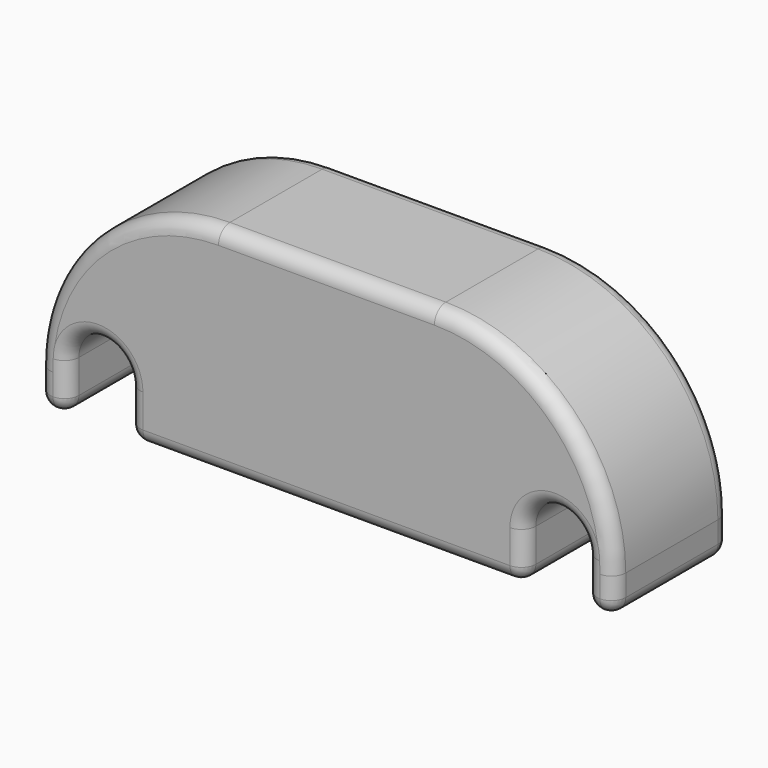
from build123d import *

# Parameters (mm, degrees)
F1_DEPTH     = 20
F2_R         = 1.99999
F3_T1_DEPTH  = 30
F3_T3_DEPTH  = 8.00001
F3_T5_DEPTH  = 10.00002
F3_T7_DEPTH  = 9.6446849121
F3_T9_DEPTH  = 61.00002
F3_T11_DEPTH = 10.00002
F3_T14_ANGLE = 90
F3_T16_ANGLE = 90
F3_T18_ANGLE = 90
F3_T20_ANGLE = 90
F3_T22_ANGLE = 180
F3_T24_ANGLE = 90
F3_T26_ANGLE = 90
F3_T28_ANGLE = 180
F3_T30_ANGLE = 90
F3_T32_ANGLE = 90
F3_T34_ANGLE = 90
F3_T36_ANGLE = 90
F3_T38_ANGLE = 90
F3_T40_ANGLE = 90
F3_T42_ANGLE = 180
F3_T44_ANGLE = 90
F3_T46_ANGLE = 90
F3_T48_ANGLE = 180
F3_T50_ANGLE = 90
F3_T52_ANGLE = 90


# Not quite as in the source:
# - a fillet or chamfer that OpenCascade refuses, or shapes differently, is made with other operations: its cross-section is extruded or revolved along the edge and cut away or added
# - a fillet or chamfer is up to 0.001 mm smaller than in the source, because OpenCascade refuses the exact size


with BuildPart() as f1:
    # F0 (on Front) → F1 (new body)
    with BuildSketch(Plane.XZ):
        with BuildLine():
            Line((15, 15), (-15, 15))
            ThreePointArc((-15, 15), (-32.6776695297, 7.6776695297), (-40, -10))
            Line((-40, -10), (-40, -15))
            Line((-40, -15), (-36, -15))
            Line((-36, -15), (-36, -8.3553250879))
            ThreePointArc((-36, -8.3553250879), (-31.75, -4.1053250879), (-27.5, -8.3553250879))
            Line((-27.5, -8.3553250879), (-27.5, -15))
            Line((-27.5, -15), (27.5, -15))
            Line((27.5, -15), (27.5, -8.3553250879))
            ThreePointArc((27.5, -8.3553250879), (31.75, -4.1053250879), (36, -8.3553250879))
            Line((36, -8.3553250879), (36, -15))
            Line((36, -15), (40, -15))
            Line((40, -15), (40, -10))
            ThreePointArc((40, -10), (32.6776695297, 7.6776695297), (15, 15))
        make_face()
    extrude(amount=F1_DEPTH)

    # F2 (radius 2 in the source; OpenCascade refuses exactly that, so slightly less here)
    f2_edges = [f1.edges().sort_by_distance(p)[0] for p in [
        (36, -10, -15),
        (27.5, -10, -15),
        (40, -10, -15),
        (-27.5, -10, -15),
        (-36, -10, -15),
        (-40, -10, -15),
    ]]
    fillet(f2_edges, radius=F2_R)

    # F3: fillet of radius 2 on 2 edges, made by hand

    # F3_s2 → F3_t1 (cut)
    with BuildSketch(Plane.YZ.offset(-15)):
        with BuildLine():
            ThreePointArc((0, 13), (-0.5857864376, 14.4142135624), (-2, 15))
            Line((-2, 15), (0, 15))
            Line((0, 15), (0, 13))
        make_face()
        with BuildLine():
            ThreePointArc((-20, 13), (-19.4142135624, 14.4142135624), (-18, 15))
            Line((-18, 15), (-20, 15))
            Line((-20, 15), (-20, 13))
        make_face()
    extrude(amount=F3_T1_DEPTH, mode=Mode.SUBTRACT)

    # F3_s4 → F3_t3 (cut)
    with BuildSketch(Plane.XY.offset(-18.00001)):
        with BuildLine():
            ThreePointArc((38, -20), (39.4142135624, -19.4142135624), (40, -18))
            Line((40, -18), (40, -20))
            Line((40, -20), (38, -20))
        make_face()
        with BuildLine():
            ThreePointArc((-40, -18), (-39.4142135624, -19.4142135624), (-38, -20))
            Line((-38, -20), (-40, -20))
            Line((-40, -20), (-40, -18))
        make_face()
        with BuildLine():
            ThreePointArc((-40, -2), (-39.4142135624, -0.5857864376), (-38, 0))
            Line((-38, 0), (-40, 0))
            Line((-40, 0), (-40, -2))
        make_face()
        with BuildLine():
            ThreePointArc((38, 0), (39.4142135624, -0.5857864376), (40, -2))
            Line((40, -2), (40, 0))
            Line((40, 0), (38, 0))
        make_face()
    extrude(amount=F3_T3_DEPTH, mode=Mode.SUBTRACT)

    # F3_s6 → F3_t5 (cut)
    with BuildSketch(Plane.YZ.offset(-43.00001)):
        with BuildLine():
            ThreePointArc((-20, -13), (-19.4142135624, -14.4142135624), (-18, -15))
            Line((-18, -15), (-20, -15))
            Line((-20, -15), (-20, -13))
        make_face()
        with BuildLine():
            ThreePointArc((0, -13), (-0.5857864376, -14.4142135624), (-2, -15))
            Line((-2, -15), (0, -15))
            Line((0, -15), (0, -13))
        make_face()
    extrude(amount=F3_T5_DEPTH, mode=Mode.SUBTRACT)

    # F3_s8 → F3_t7 (cut)
    with BuildSketch(Plane.XY.offset(-18.00001)):
        with BuildLine():
            ThreePointArc((-38, -20), (-36.5857864376, -19.4142135624), (-36, -18))
            Line((-36, -18), (-36, -20))
            Line((-36, -20), (-38, -20))
        make_face()
        with BuildLine():
            ThreePointArc((-25.5, -20), (-26.9142135624, -19.4142135624), (-27.5, -18))
            Line((-27.5, -18), (-27.5, -20))
            Line((-27.5, -20), (-25.5, -20))
        make_face()
        with BuildLine():
            ThreePointArc((25.5, -20), (26.9142135624, -19.4142135624), (27.5, -18))
            Line((27.5, -18), (27.5, -20))
            Line((27.5, -20), (25.5, -20))
        make_face()
        with BuildLine():
            ThreePointArc((38, -20), (36.5857864376, -19.4142135624), (36, -18))
            Line((36, -18), (36, -20))
            Line((36, -20), (38, -20))
        make_face()
        with BuildLine():
            ThreePointArc((-38, 0), (-36.5857864376, -0.5857864376), (-36, -2))
            Line((-36, -2), (-36, 0))
            Line((-36, 0), (-38, 0))
        make_face()
        with BuildLine():
            ThreePointArc((-25.5, 0), (-26.9142135624, -0.5857864376), (-27.5, -2))
            Line((-27.5, -2), (-27.5, 0))
            Line((-27.5, 0), (-25.5, 0))
        make_face()
        with BuildLine():
            ThreePointArc((25.5, 0), (26.9142135624, -0.5857864376), (27.5, -2))
            Line((27.5, -2), (27.5, 0))
            Line((27.5, 0), (25.5, 0))
        make_face()
        with BuildLine():
            ThreePointArc((38, 0), (36.5857864376, -0.5857864376), (36, -2))
            Line((36, -2), (36, 0))
            Line((36, 0), (38, 0))
        make_face()
    extrude(amount=F3_T7_DEPTH, mode=Mode.SUBTRACT)

    # F3_s10 → F3_t9 (cut)
    with BuildSketch(Plane.YZ.offset(-30.50001)):
        with BuildLine():
            ThreePointArc((-20, -13), (-19.4142135624, -14.4142135624), (-18, -15))
            Line((-18, -15), (-20, -15))
            Line((-20, -15), (-20, -13))
        make_face()
        with BuildLine():
            ThreePointArc((0, -13), (-0.5857864376, -14.4142135624), (-2, -15))
            Line((-2, -15), (0, -15))
            Line((0, -15), (0, -13))
        make_face()
    extrude(amount=F3_T9_DEPTH, mode=Mode.SUBTRACT)

    # F3_s12 → F3_t11 (cut)
    with BuildSketch(Plane.YZ.offset(32.99999)):
        with BuildLine():
            ThreePointArc((-20, -13), (-19.4142135624, -14.4142135624), (-18, -15))
            Line((-18, -15), (-20, -15))
            Line((-20, -15), (-20, -13))
        make_face()
        with BuildLine():
            ThreePointArc((0, -13), (-0.5857864376, -14.4142135624), (-2, -15))
            Line((-2, -15), (0, -15))
            Line((0, -15), (0, -13))
        make_face()
    extrude(amount=F3_T11_DEPTH, mode=Mode.SUBTRACT)

    # F3_s13 → F3_t14 (revolve, cut)
    with BuildSketch(Plane.XY.offset(-10)):
        with BuildLine():
            ThreePointArc((38, -20), (39.4142135624, -19.4142135624), (40, -18))
            Line((40, -18), (40, -20))
            Line((40, -20), (38, -20))
        make_face()
    revolve(axis=Axis((15, -20, -10), (0, -1, 0)), revolution_arc=F3_T14_ANGLE, mode=Mode.SUBTRACT)

    # F3_s15 → F3_t16 (revolve, cut)
    with BuildSketch(Plane.YZ.offset(-15)):
        with BuildLine():
            ThreePointArc((-18, 15), (-19.4142135624, 14.4142135624), (-20, 13))
            Line((-20, 13), (-20, 15))
            Line((-20, 15), (-18, 15))
        make_face()
    revolve(axis=Axis((-15, -20, -10), (0, -1, 0)), revolution_arc=F3_T16_ANGLE, mode=Mode.SUBTRACT)

    # F3_s17 → F3_t18 (revolve, cut)
    with BuildSketch(Plane.XY.offset(-13.00001)):
        with BuildLine():
            ThreePointArc((-40, -18), (-39.4142170979, -19.4142100268), (-38.00001, -20))
            Line((-38.00001, -20), (-40, -20))
            Line((-40, -20), (-40, -18))
        make_face()
    revolve(axis=Axis((-38.00001, -20, -13.00001), (0, -1, 0)), revolution_arc=F3_T18_ANGLE, mode=Mode.SUBTRACT)

    # F3_s19 → F3_t20 (revolve, cut)
    with BuildSketch(Plane.YZ.offset(-37.99999)):
        with BuildLine():
            ThreePointArc((-20, -13.00001), (-19.4142100268, -14.4142170979), (-18, -15))
            Line((-18, -15), (-20, -15))
            Line((-20, -15), (-20, -13.00001))
        make_face()
    revolve(axis=Axis((-37.99999, -20, -13.00001), (0, -1, 0)), revolution_arc=F3_T20_ANGLE, mode=Mode.SUBTRACT)

    # F3_s21 → F3_t22 (revolve, cut)
    with BuildSketch(Plane.XY.offset(-8.3553250879)):
        with BuildLine():
            ThreePointArc((-38, -20), (-36.5857864376, -19.4142135624), (-36, -18))
            Line((-36, -18), (-36, -20))
            Line((-36, -20), (-38, -20))
        make_face()
    revolve(axis=Axis((-31.75, -20, -8.3553250879), (0, 1, 0)), revolution_arc=F3_T22_ANGLE, mode=Mode.SUBTRACT)

    # F3_s23 → F3_t24 (revolve, cut)
    with BuildSketch(Plane.XY.offset(-13.00001)):
        with BuildLine():
            ThreePointArc((-25.50001, -20), (-26.9142170979, -19.4142100268), (-27.5, -18))
            Line((-27.5, -18), (-27.5, -20))
            Line((-27.5, -20), (-25.50001, -20))
        make_face()
    revolve(axis=Axis((-25.50001, -20, -13.00001), (0, -1, 0)), revolution_arc=F3_T24_ANGLE, mode=Mode.SUBTRACT)

    # F3_s25 → F3_t26 (revolve, cut)
    with BuildSketch(Plane.YZ.offset(25.50001)):
        with BuildLine():
            ThreePointArc((-20, -13.00001), (-19.4142100268, -14.4142170979), (-18, -15))
            Line((-18, -15), (-20, -15))
            Line((-20, -15), (-20, -13.00001))
        make_face()
    revolve(axis=Axis((25.50001, -20, -13.00001), (0, -1, 0)), revolution_arc=F3_T26_ANGLE, mode=Mode.SUBTRACT)

    # F3_s27 → F3_t28 (revolve, cut)
    with BuildSketch(Plane.XY.offset(-8.3553250879)):
        with BuildLine():
            ThreePointArc((25.5, -20), (26.9142135624, -19.4142135624), (27.5, -18))
            Line((27.5, -18), (27.5, -20))
            Line((27.5, -20), (25.5, -20))
        make_face()
    revolve(axis=Axis((31.75, -20, -8.3553250879), (0, 1, 0)), revolution_arc=F3_T28_ANGLE, mode=Mode.SUBTRACT)

    # F3_s29 → F3_t30 (revolve, cut)
    with BuildSketch(Plane.XY.offset(-13.00001)):
        with BuildLine():
            ThreePointArc((37.99999, -20), (36.5857829021, -19.4142100268), (36, -18))
            Line((36, -18), (36, -20))
            Line((36, -20), (37.99999, -20))
        make_face()
    revolve(axis=Axis((37.99999, -20, -13.00001), (0, -1, 0)), revolution_arc=F3_T30_ANGLE, mode=Mode.SUBTRACT)

    # F3_s31 → F3_t32 (revolve, cut)
    with BuildSketch(Plane.YZ.offset(38.00001)):
        with BuildLine():
            ThreePointArc((-20, -13.00001), (-19.4142100268, -14.4142170979), (-18, -15))
            Line((-18, -15), (-20, -15))
            Line((-20, -15), (-20, -13.00001))
        make_face()
    revolve(axis=Axis((38.00001, -20, -13.00001), (0, -1, 0)), revolution_arc=F3_T32_ANGLE, mode=Mode.SUBTRACT)

    # F3_s33 → F3_t34 (revolve, cut)
    with BuildSketch(Plane.XY.offset(-10)):
        with BuildLine():
            ThreePointArc((38, 0), (39.4142135624, -0.5857864376), (40, -2))
            Line((40, -2), (40, 0))
            Line((40, 0), (38, 0))
        make_face()
    revolve(axis=Axis((15, 0, -10), (0, -1, 0)), revolution_arc=F3_T34_ANGLE, mode=Mode.SUBTRACT)

    # F3_s35 → F3_t36 (revolve, cut)
    with BuildSketch(Plane.YZ.offset(-15)):
        with BuildLine():
            ThreePointArc((0, 13), (-0.5857864376, 14.4142135624), (-2, 15))
            Line((-2, 15), (0, 15))
            Line((0, 15), (0, 13))
        make_face()
    revolve(axis=Axis((-15, 0, -10), (0, -1, 0)), revolution_arc=F3_T36_ANGLE, mode=Mode.SUBTRACT)

    # F3_s37 → F3_t38 (revolve, cut)
    with BuildSketch(Plane.XY.offset(-13.00001)):
        with BuildLine():
            ThreePointArc((-38.00001, 0), (-39.4142170979, -0.5857899732), (-40, -2))
            Line((-40, -2), (-40, 0))
            Line((-40, 0), (-38.00001, 0))
        make_face()
    revolve(axis=Axis((-38.00001, 0, -13.00001), (0, -1, 0)), revolution_arc=F3_T38_ANGLE, mode=Mode.SUBTRACT)

    # F3_s39 → F3_t40 (revolve, cut)
    with BuildSketch(Plane.YZ.offset(-37.99999)):
        with BuildLine():
            ThreePointArc((0, -13.00001), (-0.5857899732, -14.4142170979), (-2, -15))
            Line((-2, -15), (0, -15))
            Line((0, -15), (0, -13.00001))
        make_face()
    revolve(axis=Axis((-37.99999, 0, -13.00001), (0, -1, 0)), revolution_arc=F3_T40_ANGLE, mode=Mode.SUBTRACT)

    # F3_s41 → F3_t42 (revolve, cut)
    with BuildSketch(Plane.XY.offset(-8.3553250879)):
        with BuildLine():
            ThreePointArc((-38, 0), (-36.5857864376, -0.5857864376), (-36, -2))
            Line((-36, -2), (-36, 0))
            Line((-36, 0), (-38, 0))
        make_face()
    revolve(axis=Axis((-31.75, 0, -8.3553250879), (0, 1, 0)), revolution_arc=F3_T42_ANGLE, mode=Mode.SUBTRACT)

    # F3_s43 → F3_t44 (revolve, cut)
    with BuildSketch(Plane.XY.offset(-13.00001)):
        with BuildLine():
            ThreePointArc((-25.50001, 0), (-26.9142170979, -0.5857899732), (-27.5, -2))
            Line((-27.5, -2), (-27.5, 0))
            Line((-27.5, 0), (-25.50001, 0))
        make_face()
    revolve(axis=Axis((-25.50001, 0, -13.00001), (0, -1, 0)), revolution_arc=F3_T44_ANGLE, mode=Mode.SUBTRACT)

    # F3_s45 → F3_t46 (revolve, cut)
    with BuildSketch(Plane.YZ.offset(25.50001)):
        with BuildLine():
            ThreePointArc((0, -13.00001), (-0.5857899732, -14.4142170979), (-2, -15))
            Line((-2, -15), (0, -15))
            Line((0, -15), (0, -13.00001))
        make_face()
    revolve(axis=Axis((25.50001, 0, -13.00001), (0, -1, 0)), revolution_arc=F3_T46_ANGLE, mode=Mode.SUBTRACT)

    # F3_s47 → F3_t48 (revolve, cut)
    with BuildSketch(Plane.XY.offset(-8.3553250879)):
        with BuildLine():
            ThreePointArc((25.5, 0), (26.9142135624, -0.5857864376), (27.5, -2))
            Line((27.5, -2), (27.5, 0))
            Line((27.5, 0), (25.5, 0))
        make_face()
    revolve(axis=Axis((31.75, 0, -8.3553250879), (0, 1, 0)), revolution_arc=F3_T48_ANGLE, mode=Mode.SUBTRACT)

    # F3_s49 → F3_t50 (revolve, cut)
    with BuildSketch(Plane.XY.offset(-13.00001)):
        with BuildLine():
            ThreePointArc((37.99999, 0), (36.5857829021, -0.5857899732), (36, -2))
            Line((36, -2), (36, 0))
            Line((36, 0), (37.99999, 0))
        make_face()
    revolve(axis=Axis((37.99999, 0, -13.00001), (0, -1, 0)), revolution_arc=F3_T50_ANGLE, mode=Mode.SUBTRACT)

    # F3_s51 → F3_t52 (revolve, cut)
    with BuildSketch(Plane.YZ.offset(38.00001)):
        with BuildLine():
            ThreePointArc((0, -13.00001), (-0.5857899732, -14.4142170979), (-2, -15))
            Line((-2, -15), (0, -15))
            Line((0, -15), (0, -13.00001))
        make_face()
    revolve(axis=Axis((38.00001, 0, -13.00001), (0, -1, 0)), revolution_arc=F3_T52_ANGLE, mode=Mode.SUBTRACT)


solid = f1.part
